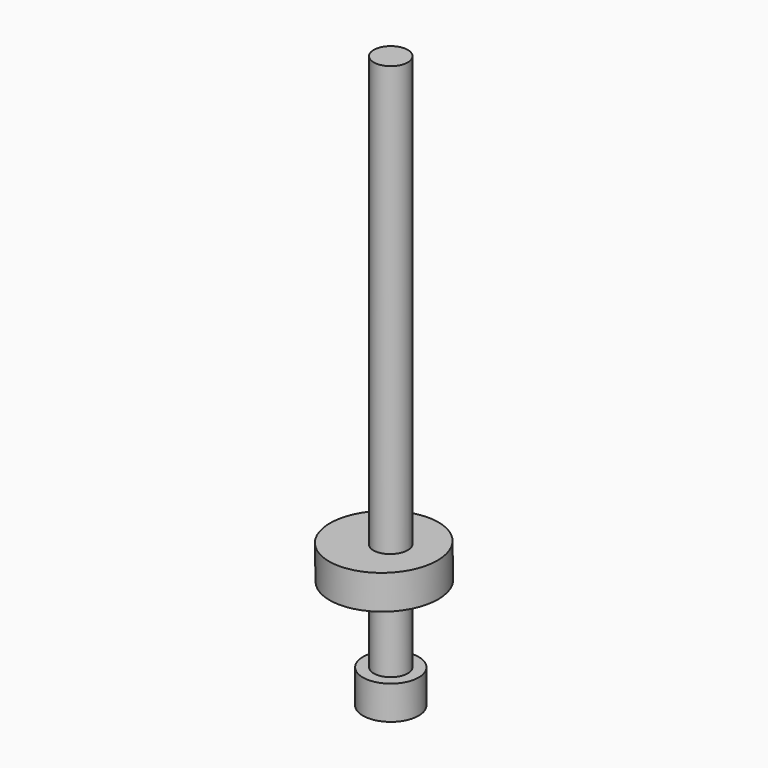
from build123d import *

# Parameters (mm, degrees)
F0_R     = 4.925
F1_DEPTH = 5.95
F2_R     = 3
F3_DEPTH = 95
F6_R     = 9.5
F7_DEPTH = 6


# Not quite as in the source:
# - a feature of the source that left no trace in its solid (it failed there, or was rolled back) is left out


with BuildPart() as f1:
    # F0 (on Top) → F1 (new body)
    with BuildSketch(Plane.XY):
        Circle(F0_R)
    extrude(amount=F1_DEPTH)

    # F2 (on face) → F3 (join)
    with BuildSketch(Plane.XY.offset(5.95)):
        Circle(F2_R)
    extrude(amount=F3_DEPTH)

    # F6 (on face) → F7 (join)
    with BuildSketch(Plane(origin=(-0.3810464275, 0, 19.0483774936), x_dir=(0.9997999772, 0, 0.0200001396), z_dir=(0.0200001396, 0, -0.9997999772))):
        with Locations((-0.7457245374, 0)):
            Circle(F6_R)
    extrude(amount=-F7_DEPTH)


solid = f1.part
